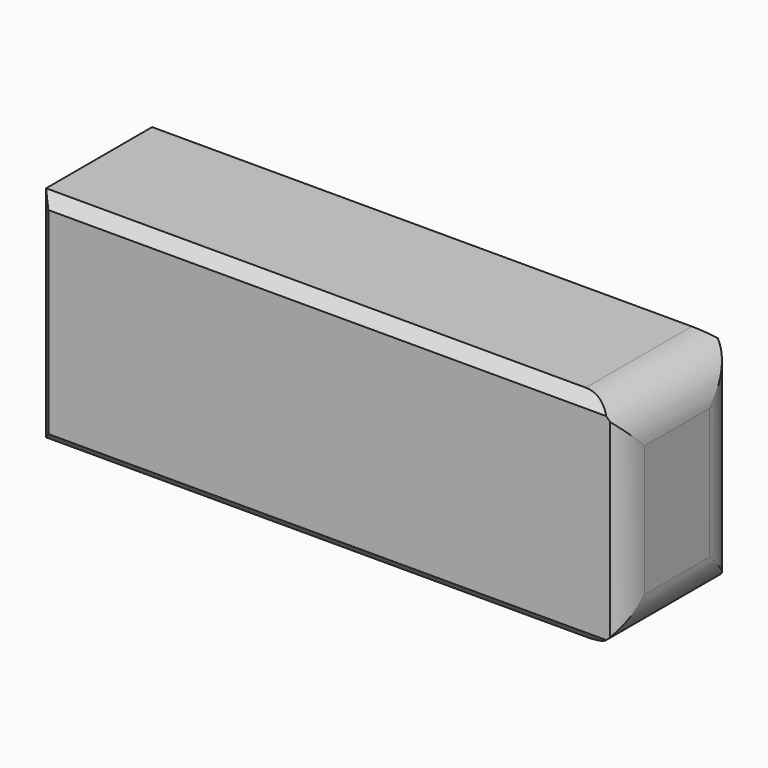
from build123d import *

# Parameters (mm, degrees)
F0_W        = 67.139275372
F0_H        = 25.2126324922
F1_DEPTH    = 8.89
F2_SIZE     = 1.27
F3_T1_DEPTH = 48.0726324922
F3_T3_DEPTH = 35.6631533174
F3_T5_DEPTH = 40.64


# Not quite as in the source:
# - a fillet or chamfer that OpenCascade refuses, or shapes differently, is made with other operations: its cross-section is extruded or revolved along the edge and cut away or added


with BuildPart() as f1:
    # F0 (on Front) → F1 (new body, symmetric)
    with BuildSketch(Plane.XZ):
        Rectangle(F0_W, F0_H)
    extrude(amount=F1_DEPTH, both=True)

    # F2
    f2_edges = [f1.edges().sort_by_distance(p)[0] for p in [
        (0, -8.89, 12.606316),
        (33.569638, -8.89, 0),
        (-33.569638, -8.89, 0),
        (0, -8.89, -12.606316),
        (0, 8.89, 12.606316),
        (0, 8.89, -12.606316),
    ]]
    chamfer(f2_edges, length=F2_SIZE)

    # F3: fillet of radius 5.08 on 6 edges, made by hand

    # F3_s2 → F3_t1 (cut)
    with BuildSketch(Plane.XY.offset(-24.0363162461)):
        with BuildLine():
            ThreePointArc((33.569637686, 3.81), (32.0817401344, 7.4021024484), (28.489637686, 8.89))
            Line((28.489637686, 8.89), (33.569637686, 8.89))
            Line((33.569637686, 8.89), (33.569637686, 3.81))
        make_face()
    extrude(amount=F3_T1_DEPTH, mode=Mode.SUBTRACT)

    # F3_s4 → F3_t3 (cut)
    with BuildSketch(Plane.XY.offset(-17.8315766587)):
        with BuildLine():
            ThreePointArc((33.569637686, -5.5298958349), (33.2415425672, -7.3259470592), (32.299637686, -8.89))
            Line((32.299637686, -8.89), (33.569637686, -7.62))
            Line((33.569637686, -7.62), (33.569637686, -5.5298958349))
        make_face()
    extrude(amount=F3_T3_DEPTH, mode=Mode.SUBTRACT)

    # F3_s6 → F3_t5 (cut)
    with BuildSketch(Plane.XZ.offset(-20.32)):
        with BuildLine():
            ThreePointArc((33.569637686, -7.5263162461), (32.0817401344, -11.1184186945), (28.489637686, -12.6063162461))
            Line((28.489637686, -12.6063162461), (33.569637686, -12.6063162461))
            Line((33.569637686, -12.6063162461), (33.569637686, -7.5263162461))
        make_face()
        with BuildLine():
            ThreePointArc((33.569637686, 7.5263162461), (32.0817401344, 11.1184186945), (28.489637686, 12.6063162461))
            Line((28.489637686, 12.6063162461), (33.569637686, 12.6063162461))
            Line((33.569637686, 12.6063162461), (33.569637686, 7.5263162461))
        make_face()
    extrude(amount=F3_T5_DEPTH, mode=Mode.SUBTRACT)


solid = f1.part
